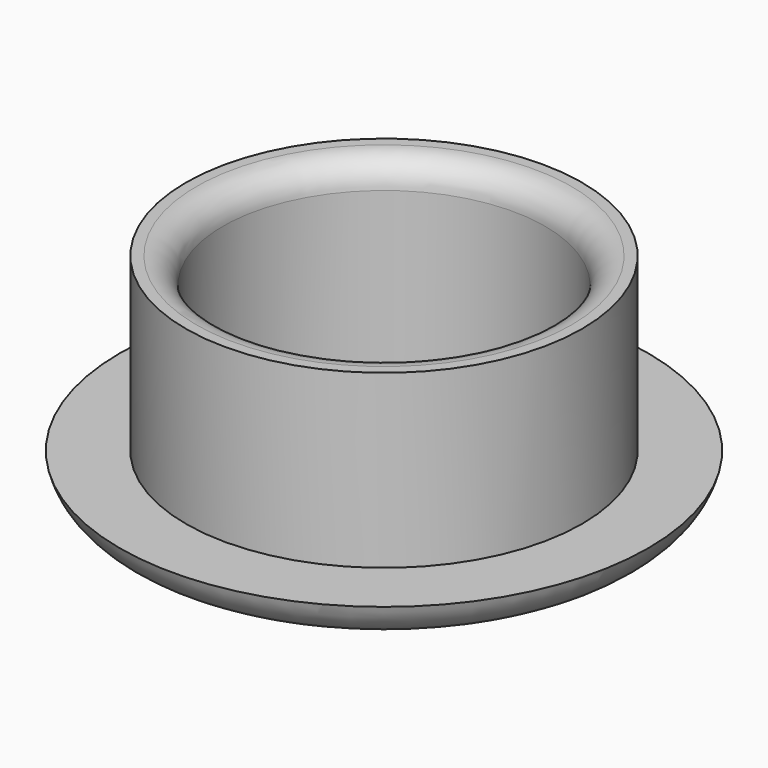
from build123d import *

# Parameters (mm, degrees)
F0_R     = 10
F0_R_2   = 7.5
F1_DEPTH = 1.5
F0_R_3   = 6.1
F2_DEPTH = 8
F4_R     = 1


# Not quite as in the source:
# - a fillet or chamfer that OpenCascade refuses, or shapes differently, is made with other operations: its cross-section is extruded or revolved along the edge and cut away or added


with BuildPart() as f1:
    # F0 (on Top) → F1 (new body)
    with BuildSketch(Plane.XY):
        Circle(F0_R)
        Circle(F0_R_2, mode=Mode.SUBTRACT)
    extrude(amount=F1_DEPTH)

    # F0 (on Top) → F2 (join)
    with BuildSketch(Plane.XY):
        Circle(F0_R_2)
        Circle(F0_R_3, mode=Mode.SUBTRACT)
    extrude(amount=F2_DEPTH)

    # F3: fillet of radius 2 on 1 edges, made by hand

    # F3_s1 → F3_t2 (revolve, cut)
    with BuildSketch(Plane.XZ):
        with BuildLine():
            ThreePointArc((10, 1.5), (9.2882531983, 0.4188611699), (8.0635083269, 0))
            Line((8.0635083269, 0), (10, 0))
            Line((10, 0), (10, 1.5))
        make_face()
    revolve(axis=Axis((0, 0, 0), (0, 0, 1)), mode=Mode.SUBTRACT)

    # F4
    f4_edges = [f1.edges().sort_by_distance(p)[0] for p in [
        (-6.1, 0, 8),
    ]]
    fillet(f4_edges, radius=F4_R)


solid = f1.part
